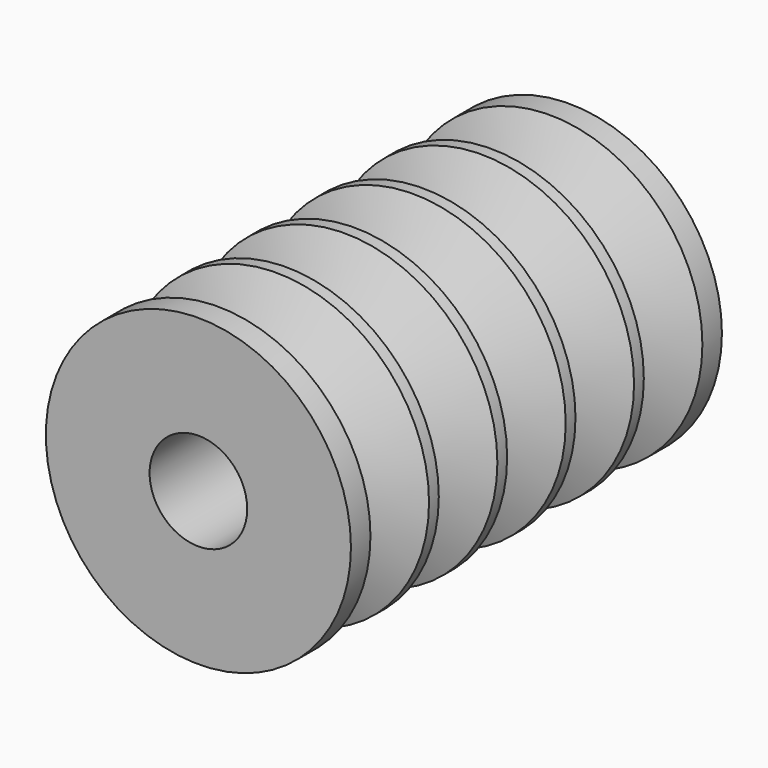
from build123d import *

# Parameters (mm, degrees)
F0_R      = 12.5
F1_DEPTH  = 5
F2_SIZE2  = 6.4335207615
F2_SIZE   = 3
F3_R      = 12.5
F4_DEPTH  = 7
F5_SIZE2  = 6.433511
F5_SIZE   = 2.99999
F6_R      = 12.5
F7_DEPTH  = 7
F8_SIZE2  = 6.433421
F8_SIZE   = 2.9999
F9_R      = 12.5
F10_DEPTH = 7
F11_SIZE2 = 6.432521
F11_SIZE  = 2.999
F12_R     = 12.5
F13_DEPTH = 7
F15_R     = 12.5
F16_DEPTH = 5
F17_SIZE2 = 6.433511
F17_SIZE  = 2.99999
F19_D     = 8


# Not quite as in the source:
# - a fillet or chamfer that OpenCascade refuses, or shapes differently, is made with other operations: its cross-section is extruded or revolved along the edge and cut away or added
# - a fillet or chamfer is up to 0.001 mm smaller than in the source, because OpenCascade refuses the exact size


with BuildPart() as f1:
    # F0 (on Front) → F1 (new body)
    with BuildSketch(Plane.XZ):
        Circle(F0_R)
    extrude(amount=F1_DEPTH)

    # F2
    f2_edges = [f1.edges().sort_by_distance(p)[0] for p in [
        (-12.5, -5, 0),
    ]]
    f2_side = f1.faces().sort_by_distance((-12.5, -2.5, 0))[0]
    chamfer(f2_edges, length=F2_SIZE, length2=F2_SIZE2, reference=f2_side)

    # F3 (on face) → F4 (join)
    with BuildSketch(Plane.XZ.offset(5)):
        Circle(F3_R)
    extrude(amount=F4_DEPTH)

    # F5 (size 3 and 6.4335207615 in the source; OpenCascade refuses exactly that, so slightly less here)
    f5_edges = [f1.edges().sort_by_distance(p)[0] for p in [
        (-12.5, -5, 0),
        (-12.5, -12, 0),
    ]]
    f5_side = f1.faces().sort_by_distance((-12.5, -8.5, 0))[0]
    chamfer(f5_edges, length=F5_SIZE, length2=F5_SIZE2, reference=f5_side)

    # F6 (on face) → F7 (join)
    with BuildSketch(Plane.XZ.offset(12)):
        Circle(F6_R)
    extrude(amount=F7_DEPTH)

    # F8 (size 3 and 6.4335207615 in the source; OpenCascade refuses exactly that, so slightly less here)
    f8_edges = [f1.edges().sort_by_distance(p)[0] for p in [
        (-12.5, -12, 0),
        (-12.5, -19, 0),
    ]]
    f8_side = f1.faces().sort_by_distance((-12.5, -15.5, 0))[0]
    chamfer(f8_edges, length=F8_SIZE, length2=F8_SIZE2, reference=f8_side)

    # F9 (on face) → F10 (join)
    with BuildSketch(Plane.XZ.offset(19)):
        Circle(F9_R)
    extrude(amount=F10_DEPTH)

    # F11 (size 3 and 6.4335207615 in the source; OpenCascade refuses exactly that, so slightly less here)
    f11_edges = [f1.edges().sort_by_distance(p)[0] for p in [
        (-12.5, -19, 0),
        (-12.5, -26, 0),
    ]]
    f11_side = f1.faces().sort_by_distance((-12.5, -22.5, 0))[0]
    chamfer(f11_edges, length=F11_SIZE, length2=F11_SIZE2, reference=f11_side)

    # F12 (on face) → F13 (join)
    with BuildSketch(Plane.XZ.offset(26)):
        Circle(F12_R)
    extrude(amount=F13_DEPTH)

    # F14: chamfer of 3 x 6.4335207615 on 2 edges, made by hand

    # F14_s1 → F14_t2 (revolve, cut)
    with BuildSketch(Plane.XY):
        Polygon((12.5, -29), (6.0664792385, -26), (12.5, -26), align=None)
    revolve(axis=Axis((0, -26, 0), (0, -1, 0)), mode=Mode.SUBTRACT)

    # F14_s3 → F14_t4 (revolve, cut)
    with BuildSketch(Plane.XY):
        Polygon((12.5, -30), (6.0664792385, -33), (12.5, -33), align=None)
    revolve(axis=Axis((0, -33, 0), (0, -1, 0)), mode=Mode.SUBTRACT)

    # F15 (on face) → F16 (join)
    with BuildSketch(Plane.XZ.offset(33)):
        Circle(F15_R)
    extrude(amount=F16_DEPTH)

    # F17 (size 3 and 6.4335207615 in the source; OpenCascade refuses exactly that, so slightly less here)
    f17_edges = [f1.edges().sort_by_distance(p)[0] for p in [
        (-12.5, -33, 0),
    ]]
    f17_side = f1.faces().sort_by_distance((-12.5, -35.5, 0))[0]
    chamfer(f17_edges, length=F17_SIZE, length2=F17_SIZE2, reference=f17_side)

    # F19 (through all)
    with Locations(Plane(origin=(0, 0, 0), x_dir=(-1, 0, 0), z_dir=(0, 1, 0))):
        with Locations((0, 0)):
            Hole(F19_D / 2)


solid = f1.part
